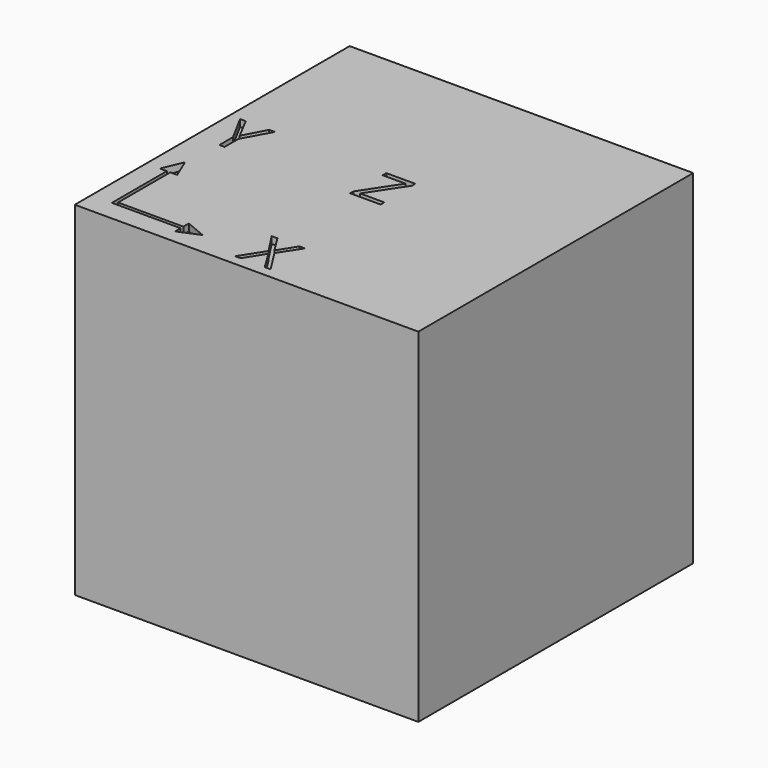
from build123d import *

# Parameters (mm, degrees)
F0_W         = 100
F0_H         = 100
F1_DEPTH     = 100
F2_TEXT_SIZE = 18.0555555556
F3_DEPTH     = 2


# Not quite as in the source:
# - Text() gives the source's letters only with a copy of the font that has no kerning and outlines rounded to 1/6400 em; it was checked with that copy


with BuildPart() as f1:
    # F0 (on Top) → F1 (new body)
    with BuildSketch(Plane.XY):
        with Locations((-11.603783071, 18.7621183693)):
            Rectangle(F0_W, F0_H)
    extrude(amount=F1_DEPTH)

    # F2 (on face) → F3 (cut)
    with BuildSketch(Plane.XY.offset(100)):
        Polygon((-55.603783071, -5.2378816307), (-55.603783071, -25.2378816307), (-35.603783071, -25.2378816307), (-35.603783071, -27.2378816307), (-29.603783071, -24.7378816307), (-35.603783071, -22.2378816307), (-35.603783071, -24.2378816307), (-54.603783071, -24.2378816307), (-54.603783071, -5.2378816307), (-52.603783071, -5.2378816307), (-55.103783071, 0.7621183693), (-57.603783071, -5.2378816307), align=None)
        with Locations((-17.3646337655, -28.2378816307)):
            Text('X', F2_TEXT_SIZE, font='Open Sans', text_align=(TextAlign.LEFT, TextAlign.BOTTOM))
        with Locations((-58.603783071, 12.2621183693)):
            Text('Y', F2_TEXT_SIZE, font='Open Sans', text_align=(TextAlign.LEFT, TextAlign.BOTTOM))
        with Locations((-16.9809532099, 12.2621183693)):
            Text('Z', F2_TEXT_SIZE, font='Open Sans', text_align=(TextAlign.LEFT, TextAlign.BOTTOM))
    extrude(amount=-F3_DEPTH, mode=Mode.SUBTRACT)


solid = f1.part
